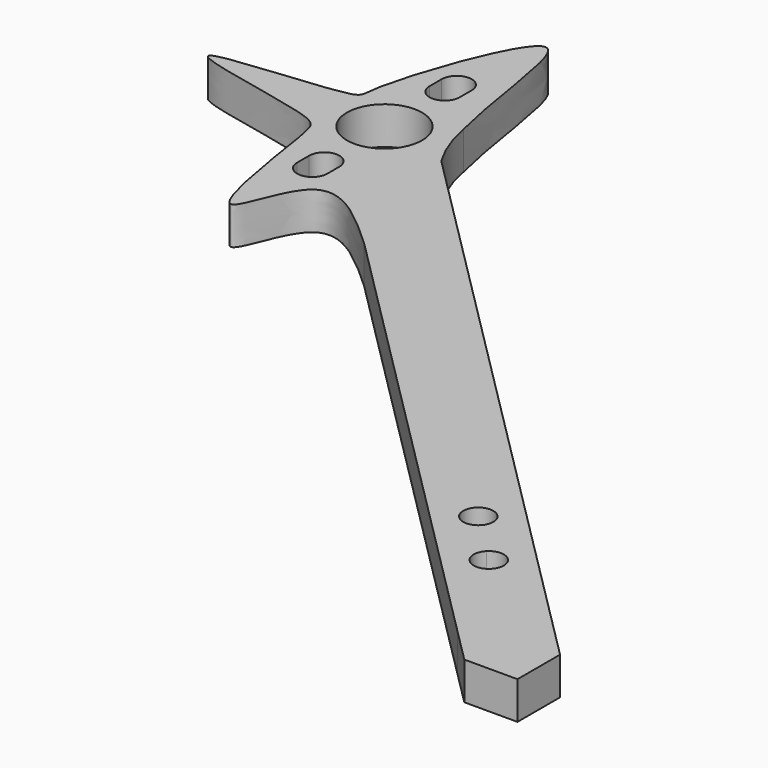
from build123d import *

# Parameters (mm, degrees)
F0_R     = 3.9999976597
F1_DEPTH = 4


with BuildPart() as f1:
    # F0 (on Top) → F1 (new body)
    with BuildSketch(Plane.XY):
        with BuildLine():
            Line((7.7150141945, 1.9408052288), (4.1794802266, 5.4763390728))
            Line((4.1794802266, 5.4763390728), (-45.8945933996, 55.5504109444))
            Line((-45.8945933996, 55.5504109444), (-49.0424586571, 58.6982760916))
            add(Edge.make_bspline(
                [(-49.0424586571, 58.6982760917), (-50.8783960205, 60.0346249378), (-53.4866069413, 61.6986557194), (-55.4321902376, 65.0880074483)],
                knots=[0.0630834581, 0.0630834581, 0.0630834581, 0.0630834581, 0.1366310285, 0.1366310285, 0.1366310285, 0.1366310285], degree=3))
            ThreePointArc((-55.4321902376, 65.0880074483), (-56.7541503558, 67.7893938967), (-57.5552814645, 70.6882309471))
            add(Edge.make_bspline(
                [(-57.5552814645, 70.6882309471), (-59.3304430199, 77.6921116304), (-60.0829814446, 96.3208412506), (-68.6570351686, 71.4284700086), (-67.2064852054, 69.2081633345), (-92.3914116748, 68.3586081886), (-68.6432624157, 64.8740884961), (-67.4455031945, 62.6782310544), (-66.7213225211, 56.2991866457), (-64.1719257131, 43.6209538428), (-61.2499457456, 58.7746168707), (-54.7179806248, 52.7710993697), (-51.1458562022, 49.4879661793)],
                knots=[0.1694455517, 0.1694455517, 0.1694455517, 0.1694455517, 0.2755113584, 0.3870974654, 0.4299282501, 0.5331299784, 0.6347488857, 0.6806016142, 0.7553172113, 0.8333688983, 0.9088747388, 1, 1, 1, 1], degree=3))
            Line((-51.1458562022, 49.4879661793), (-1.4773740234, -0.1805142459))
            Line((-1.4773740234, -0.1805142459), (2.058159945, -3.7160480894))
            Line((2.058159945, -3.7160480894), (7.7150141945, -3.7160480894))
            Line((7.7150141945, -3.7160480894), (7.7150141945, 1.9408052288))
        make_face()
        with BuildLine():
            ThreePointArc((-6.4036174491, 10.4025831555), (-8.6663591489, 10.4025831156), (-8.6663591888, 12.6653248154))
            ThreePointArc((-8.6663591888, 12.6653248154), (-6.9226948402, 13.0121612429), (-5.934988319, 11.5339539854))
            ThreePointArc((-5.934988319, 11.5339539854), (-6.0567810615, 10.9216605067), (-6.4036174491, 10.4025831555))
        make_face(mode=Mode.SUBTRACT)
        with BuildLine():
            ThreePointArc((-11.9820395129, 15.9810050224), (-14.5916176402, 17.724669331), (-11.5134103828, 17.1123758523))
            ThreePointArc((-11.5134103828, 17.1123758523), (-11.6352031253, 16.5000823736), (-11.9820395129, 15.9810050224))
        make_face(mode=Mode.SUBTRACT)
        with BuildLine():
            ThreePointArc((-61.3956648634, 57.3946300292), (-62.9956648634, 55.7946300292), (-64.5956648634, 57.3946300292))
            Line((-64.5956648634, 57.3946300292), (-64.5956648634, 58.9946300292))
            ThreePointArc((-64.5956648634, 58.9946300292), (-62.9956648634, 60.5946300292), (-61.3956648634, 58.9946300292))
            Line((-61.3956648634, 58.9946300292), (-61.3956648634, 57.3946300292))
        make_face(mode=Mode.SUBTRACT)
        with Locations((-62.9956639242, 66.9946300292)):
            Circle(F0_R, mode=Mode.SUBTRACT)
        with BuildLine():
            ThreePointArc((-64.5956648634, 76.5946300292), (-62.9956648634, 78.1946300292), (-61.3956648634, 76.5946300292))
            Line((-61.3956648634, 76.5946300292), (-61.3956648634, 74.9946300292))
            ThreePointArc((-61.3956648634, 74.9946300292), (-62.9956648634, 73.3946300292), (-64.5956648634, 74.9946300292))
            Line((-64.5956648634, 74.9946300292), (-64.5956648634, 76.5946300292))
        make_face(mode=Mode.SUBTRACT)
        with BuildLine():
            add(Edge.make_bspline(
                [(-49.0424586571, 58.6982760917), (-50.8783960205, 60.0346249378), (-53.4866069413, 61.6986557194), (-55.4321902376, 65.0880074483)],
                knots=[0.0630834581, 0.0630834581, 0.0630834581, 0.0630834581, 0.1366310285, 0.1366310285, 0.1366310285, 0.1366310285], degree=3))
            Line((-49.0424586571, 58.6982760916), (-55.4321902376, 65.0880074483))
        make_face()
    extrude(amount=F1_DEPTH)


solid = f1.part
